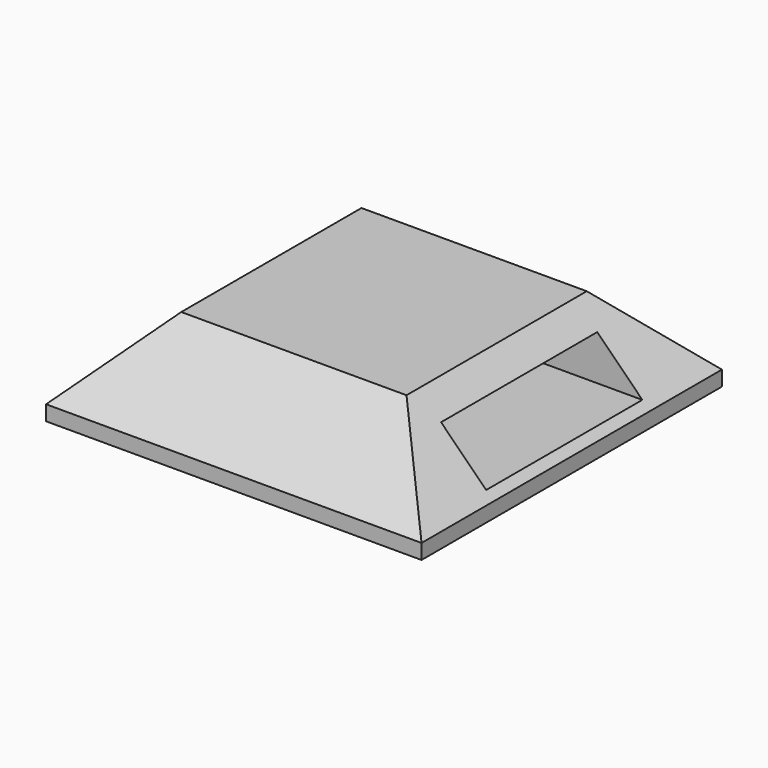
from build123d import *

# Parameters (mm, degrees)
F0_W        = 25
F0_H        = 25
F1_DEPTH    = 6
F2_W        = 13
F2_H        = 3
F3_DEPTH    = 25
F4_T1_DEPTH = 50.7168298797
F4_T3_DEPTH = 50.7168298797


# Not quite as in the source:
# - a fillet or chamfer that OpenCascade refuses, or shapes differently, is made with other operations: its cross-section is extruded or revolved along the edge and cut away or added


with BuildPart() as f1:
    # F0 (on Top) → F1 (new body)
    with BuildSketch(Plane.XY):
        with Locations((-12.5, 12.5)):
            Rectangle(F0_W, F0_H)
    extrude(amount=F1_DEPTH)

    # F2 (on face) → F3 (cut)
    with BuildSketch(Plane(origin=(-25, 0, 0), x_dir=(0, -1, 0), z_dir=(-1, 0, 0))):
        with Locations((-12.5, 3)):
            Rectangle(F2_W, F2_H)
    extrude(amount=-F3_DEPTH, mode=Mode.SUBTRACT)

    # F4: chamfer of 5 on 4 edges, made by hand

    # F4_s2 → F4_t1 (cut)
    with BuildSketch(Plane.YZ.offset(-37.8584149398)):
        Polygon((0, 1), (5, 6), (0, 6), align=None)
        Polygon((20, 6), (25, 1), (25, 6), align=None)
    extrude(amount=F4_T1_DEPTH, mode=Mode.SUBTRACT)

    # F4_s4 → F4_t3 (cut)
    with BuildSketch(Plane.XZ.offset(-37.8584149398)):
        Polygon((-25, 1), (-20, 6), (-25, 6), align=None)
        Polygon((0, 1), (-5, 6), (0, 6), align=None)
    extrude(amount=F4_T3_DEPTH, mode=Mode.SUBTRACT)


solid = f1.part
